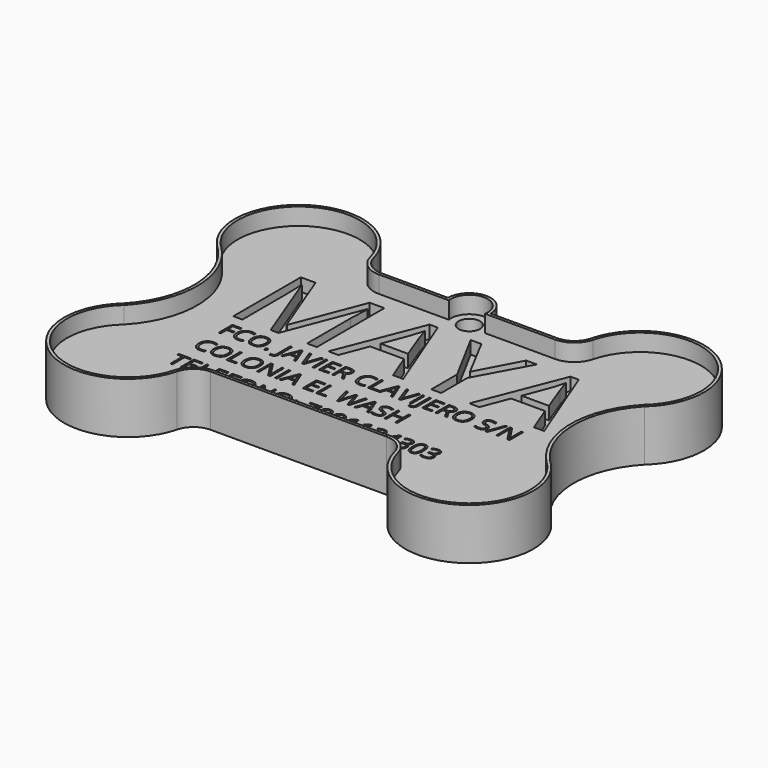
from build123d import *

# Parameters (mm, degrees)
F0_R         = 2.5
F1_DEPTH     = 8
F2_TEXT_SIZE = 27.697940661
F3_DEPTH     = 3
F5_DEPTH     = 4
F6_TEXT_SIZE = 5.5555555556
F7_DEPTH     = 4
F8_W         = 27.0967744291
F8_H         = 7.8326575458
F8_W_2       = 69.6471799165
F8_H_2       = 12.2782327235
F9_DEPTH     = 5


# Not quite as in the source:
# - Text() gives the source's letters only with a copy of the font that has no kerning and outlines rounded to 1/6400 em; it was checked with that copy


with BuildPart() as f1:
    # F0 (on Top) → F1 (new body)
    with BuildSketch(Plane.XY):
        with BuildLine():
            Line((7.1869715303, 26.1201031506), (-8.4481117386, 26.1201031506))
            ThreePointArc((-8.4481117386, 26.1201031506), (-11.5099739171, 27.1672560754), (-13.2893409214, 29.8701031506))
            ThreePointArc((-13.2893409214, 29.8701031506), (-35.6133297169, 38.9324136547), (-37.8130284697, 14.9397632631))
            ThreePointArc((-37.8130284697, 14.9397632631), (-32.2704485153, 1.1201031506), (-37.8130284697, -12.6995569619))
            ThreePointArc((-37.8130284697, -12.6995569619), (-35.6133297169, -36.6922073534), (-13.2893409214, -27.6298968494))
            ThreePointArc((-13.2893409214, -27.6298968494), (-11.5099739171, -24.9270497742), (-8.4481117386, -23.8798968494))
            Line((-8.4481117386, -23.8798968494), (32.8220547993, -23.8798968494))
            ThreePointArc((32.8220547993, -23.8798968494), (35.8839169778, -24.9270497742), (37.663283982, -27.6298968494))
            ThreePointArc((37.663283982, -27.6298968494), (59.9872727776, -36.6922073534), (62.1869715303, -12.6995569619))
            ThreePointArc((62.1869715303, -12.6995569619), (56.6443915759, 1.1201031506), (62.1869715303, 14.9397632631))
            ThreePointArc((62.1869715303, 14.9397632631), (59.9872727776, 38.9324136547), (37.663283982, 29.8701031506))
            ThreePointArc((37.663283982, 29.8701031506), (35.8839169778, 27.1672560754), (32.8220547993, 26.1201031506))
            Line((32.8220547993, 26.1201031506), (17.1869715303, 26.1201031506))
            ThreePointArc((17.1869715303, 26.1201031506), (12.1869715303, 31.1201031506), (7.1869715303, 26.1201031506))
        make_face()
        with Locations((12.1869715303, 26.1201031506)):
            Circle(F0_R, mode=Mode.SUBTRACT)
    extrude(amount=F1_DEPTH)

    # F2 (on face) → F3 (cut)
    with BuildSketch(Plane.XY.offset(8)):
        with Locations((-26.4515727758, 1.8703314709)):
            Text('MAYA', F2_TEXT_SIZE, font='Open Sans', text_align=(TextAlign.LEFT, TextAlign.BOTTOM))
    extrude(amount=-F3_DEPTH, mode=Mode.SUBTRACT)

    # F4 (on face) → F5 (join)
    with BuildSketch(Plane.XY.offset(8)):
        with BuildLine():
            ThreePointArc((-37.8130284697, -12.6995569619), (-35.6133297169, -36.6922073534), (-13.2893409214, -27.6298968494))
            ThreePointArc((-13.2893409214, -27.6298968494), (-11.5099739171, -24.9270497742), (-8.4481117386, -23.8798968494))
            Line((-8.4481117386, -23.8798968494), (32.8220547993, -23.8798968494))
            ThreePointArc((32.8220547993, -23.8798968494), (35.8839169778, -24.9270497742), (37.663283982, -27.6298968494))
            ThreePointArc((37.663283982, -27.6298968494), (59.9872727776, -36.6922073534), (62.1869715303, -12.6995569619))
            ThreePointArc((62.1869715303, -12.6995569619), (56.6443915759, 1.1201031506), (62.1869715303, 14.9397632631))
            ThreePointArc((62.1869715303, 14.9397632631), (59.9872727776, 38.9324136547), (37.663283982, 29.8701031506))
            ThreePointArc((37.663283982, 29.8701031506), (35.8839169778, 27.1672560754), (32.8220547993, 26.1201031506))
            Line((32.8220547993, 26.1201031506), (17.1869715303, 26.1201031506))
            ThreePointArc((17.1869715303, 26.1201031506), (12.1869715303, 31.1201031506), (7.1869715303, 26.1201031506))
            Line((7.1869715303, 26.1201031506), (-8.4481117386, 26.1201031506))
            ThreePointArc((-8.4481117386, 26.1201031506), (-11.5099739171, 27.1672560754), (-13.2893409214, 29.8701031506))
            ThreePointArc((-13.2893409214, 29.8701031506), (-35.6133297169, 38.9324136547), (-37.8130284697, 14.9397632631))
            ThreePointArc((-37.8130284697, 14.9397632631), (-32.2704485153, 1.1201031506), (-37.8130284697, -12.6995569619))
        make_face()
        with BuildLine():
            ThreePointArc((61.7002912634, -13.2034392133), (59.6347133107, -36.0873184597), (38.3410560676, -27.4548968494))
            ThreePointArc((38.3410560676, -27.4548968494), (36.3125776827, -24.3736511837), (32.8220547993, -23.1798968494))
            Line((32.8220547993, -23.1798968494), (-8.4481117386, -23.1798968494))
            ThreePointArc((-8.4481117386, -23.1798968494), (-11.9386346221, -24.3736511837), (-13.967113007, -27.4548968494))
            ThreePointArc((-13.967113007, -27.4548968494), (-35.2607702501, -36.0873184597), (-37.3263482028, -13.2034392133))
            ThreePointArc((-37.3263482028, -13.2034392133), (-31.5704485153, 1.1201031506), (-37.3263482028, 15.4436455145))
            ThreePointArc((-37.3263482028, 15.4436455145), (-35.2607702501, 38.3275247609), (-13.967113007, 29.6951031506))
            ThreePointArc((-13.967113007, 29.6951031506), (-11.9386346221, 26.6138574849), (-8.4481117386, 25.4201031506))
            Line((-8.4481117386, 25.4201031506), (7.9443308432, 25.4201031506))
            ThreePointArc((7.9443308432, 25.4201031506), (12.1869715303, 30.4201031506), (16.4296122174, 25.4201031506))
            Line((16.4296122174, 25.4201031506), (32.8220547993, 25.4201031506))
            ThreePointArc((32.8220547993, 25.4201031506), (36.3125776827, 26.6138574849), (38.3410560676, 29.6951031506))
            ThreePointArc((38.3410560676, 29.6951031506), (59.6347133107, 38.3275247609), (61.7002912634, 15.4436455145))
            ThreePointArc((61.7002912634, 15.4436455145), (55.9443915759, 1.1201031506), (61.7002912634, -13.2034392133))
        make_face(mode=Mode.SUBTRACT)
    extrude(amount=F5_DEPTH)

    # F6 (on face) → F7 (cut)
    with BuildSketch(Plane.XY.offset(8)):
        with Locations((-22.2876826049, -4.881355988)):
            Text('FCO. JAVIER CLAVIJERO S/N', F6_TEXT_SIZE, font='Open Sans', text_align=(TextAlign.LEFT, TextAlign.BOTTOM))
        with Locations((-22.2876826049, -12.4369115436)):
            Text('COLONIA EL WASH', F6_TEXT_SIZE, font='Open Sans', text_align=(TextAlign.LEFT, TextAlign.BOTTOM))
        with Locations((-22.2876826049, -19.9924670992)):
            Text('TELEFONO: 7891124303', F6_TEXT_SIZE, font='Open Sans', text_align=(TextAlign.LEFT, TextAlign.BOTTOM))
    extrude(amount=-F7_DEPTH, mode=Mode.SUBTRACT)

    # F8 (on Top) → F9 (cut)
    with BuildSketch(Plane.XY):
        with Locations((-56.3104841858, -46.1491961032)):
            Rectangle(F8_W, F8_H)
        with Locations((10.0554442033, -61.9203653187)):
            Rectangle(F8_W_2, F8_H_2)
        Polygon((0.6036563573, -65.7308474183), (-0.0532917555, -65.7308474183), (-0.7329344395, -63.9953099494), (-2.9199744297, -63.9953099494), (-3.5912559559, -65.7308474183), (-4.2338706553, -65.7308474183), (-2.076691943, -60.2507057063), (-1.542772295, -60.2507057063), align=None, mode=Mode.SUBTRACT)
        with BuildLine():
            Line((4.2801768868, -65.7308474183), (3.7689518099, -65.7308474183))
            Line((3.7689518099, -65.7308474183), (1.9175525829, -60.8933204057))
            Line((1.9175525829, -60.8933204057), (1.8876913051, -60.8933204057))
            add(Edge.make_bspline(
                [(1.8876913051, -60.8933204057), (1.9402471541, -61.4678513917), (1.9402471541, -62.2597724804)],
                knots=[0, 0, 0, 1, 1, 1], degree=2))
            Line((1.9402471541, -62.2597724804), (1.9402471541, -65.7308474183))
            Line((1.9402471541, -65.7308474183), (1.353771657, -65.7308474183))
            Line((1.353771657, -65.7308474183), (1.353771657, -60.2734002775))
            Line((1.353771657, -60.2734002775), (2.3093325484, -60.2734002775))
            Line((2.3093325484, -60.2734002775), (4.0377033106, -64.7752865269))
            Line((4.0377033106, -64.7752865269), (4.0675645885, -64.7752865269))
            Line((4.0675645885, -64.7752865269), (5.8102687641, -60.2734002775))
            Line((5.8102687641, -60.2734002775), (6.7586629488, -60.2734002775))
            Line((6.7586629488, -60.2734002775), (6.7586629488, -65.7308474183))
            Line((6.7586629488, -65.7308474183), (6.1244094072, -65.7308474183))
            Line((6.1244094072, -65.7308474183), (6.1244094072, -62.2143833381))
            add(Edge.make_bspline(
                [(6.1244094072, -62.2143833381), (6.1244094072, -61.6099910743), (6.1769652562, -60.9004871124)],
                knots=[0, 0, 0, 1, 1, 1], degree=2))
            Line((6.1769652562, -60.9004871124), (6.1471039783, -60.9004871124))
            Line((6.1471039783, -60.9004871124), (4.2801768868, -65.7308474183))
        make_face(mode=Mode.SUBTRACT)
        with BuildLine():
            add(Edge.make_bspline(
                [(12.3319718477, -60.9339317436), (12.9925033139, -61.68046369), (12.9925033139, -62.9943599156)],
                knots=[0, 0, 0, 1, 1, 1], degree=2))
            add(Edge.make_bspline(
                [(12.9925033139, -62.9943599156), (12.9925033139, -64.3046727879), (12.3295829455, -65.0553853132)],
                knots=[0, 0, 0, 1, 1, 1], degree=2))
            add(Edge.make_bspline(
                [(12.3295829455, -65.0553853132), (11.6666625771, -65.8060978385), (10.4877393274, -65.8060978385)],
                knots=[0, 0, 0, 1, 1, 1], degree=2))
            add(Edge.make_bspline(
                [(10.4877393274, -65.8060978385), (9.2825381532, -65.8060978385), (8.627381717, -65.0685242755)],
                knots=[0, 0, 0, 1, 1, 1], degree=2))
            add(Edge.make_bspline(
                [(8.627381717, -65.0685242755), (7.9722252809, -64.3309507124), (7.9722252809, -62.987193209)],
                knots=[0, 0, 0, 1, 1, 1], degree=2))
            add(Edge.make_bspline(
                [(7.9722252809, -62.987193209), (7.9722252809, -61.6541857655), (8.6291733937, -60.9207927814)],
                knots=[0, 0, 0, 1, 1, 1], degree=2))
            add(Edge.make_bspline(
                [(8.6291733937, -60.9207927814), (9.2861215065, -60.1873997972), (10.4949060341, -60.1873997972)],
                knots=[0, 0, 0, 1, 1, 1], degree=2))
            add(Edge.make_bspline(
                [(10.4949060341, -60.1873997972), (11.6714403816, -60.1873997972), (12.3319718477, -60.9339317436)],
                knots=[0, 0, 0, 1, 1, 1], degree=2))
        make_face(mode=Mode.SUBTRACT)
        with BuildLine():
            Line((15.9822144528, -63.4613903013), (14.8427080898, -63.4613903013))
            Line((14.8427080898, -63.4613903013), (14.8427080898, -65.7308474183))
            Line((14.8427080898, -65.7308474183), (14.2084545482, -65.7308474183))
            Line((14.2084545482, -65.7308474183), (14.2084545482, -60.2734002775))
            Line((14.2084545482, -60.2734002775), (15.7051017943, -60.2734002775))
            add(Edge.make_bspline(
                [(15.7051017943, -60.2734002775), (16.7096351813, -60.2734002775), (17.1892073037, -60.6580135362)],
                knots=[0, 0, 0, 1, 1, 1], degree=2))
            add(Edge.make_bspline(
                [(17.1892073037, -60.6580135362), (17.6687794261, -61.042626795), (17.6687794261, -61.8154366659)],
                knots=[0, 0, 0, 1, 1, 1], degree=2))
            add(Edge.make_bspline(
                [(17.6687794261, -61.8154366659), (17.6687794261, -62.8976093754), (16.5710788521, -63.2786392808)],
                knots=[0, 0, 0, 1, 1, 1], degree=2))
            Line((16.5710788521, -63.2786392808), (18.0533926848, -65.7308474183))
            Line((18.0533926848, -65.7308474183), (17.3032773851, -65.7308474183))
            Line((17.3032773851, -65.7308474183), (15.9822144528, -63.4613903013))
        make_face(mode=Mode.SUBTRACT)
    extrude(amount=F9_DEPTH, mode=Mode.SUBTRACT)


solid = f1.part
